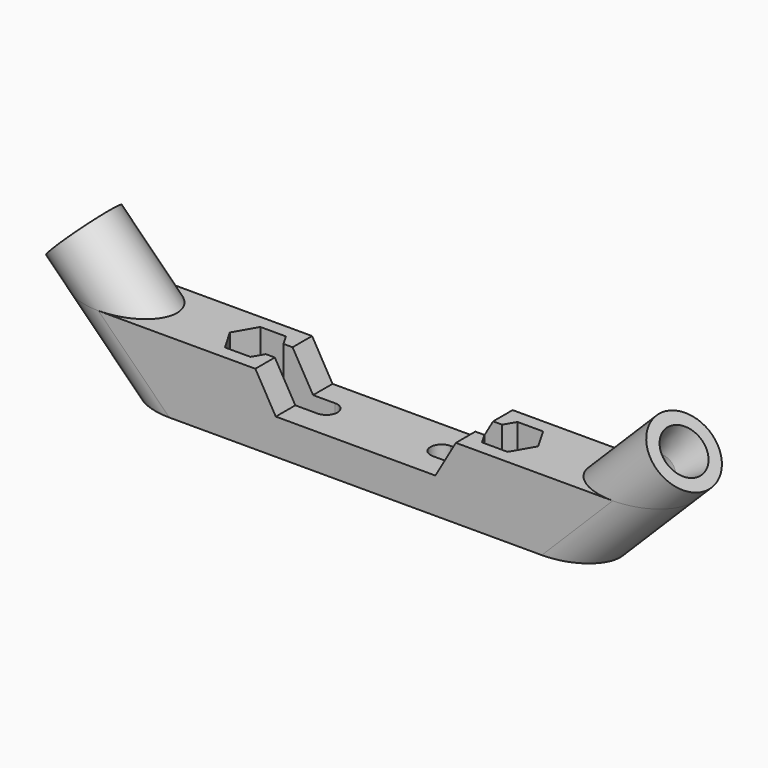
from build123d import *

# Parameters (mm, degrees)
F1_DEPTH  = 4
F2_R      = 3.99999
F4_DEPTH  = 8
F6_DEPTH  = 12.5
F9_R      = 4
F10_DEPTH = 6.851053331
F12_SIZE2 = 1
F12_SIZE  = 3.7320508076
F14_DEPTH = 8.001


# Not quite as in the source:
# - a fillet or chamfer is up to 0.001 mm smaller than in the source, because OpenCascade refuses the exact size


with BuildPart() as f1:
    # F0 (on Front) → F1 (new body, symmetric)
    with BuildSketch(Plane.XZ):
        Polygon((-26.6568542495, 0), (0, 0), (0, 8), (-34.6568542495, 8), align=None)
    extrude(amount=F1_DEPTH, both=True)

    # F2 (radius 4 in the source; OpenCascade refuses exactly that, so slightly less here)
    f2_edges = [f1.edges().sort_by_distance(p)[0] for p in [
        (-30.656854, 4, 4),
        (-30.656854, -4, 4),
    ]]
    fillet(f2_edges, radius=F2_R)

    # F3 (on face) → F4 (cut, through all)
    with BuildSketch(Plane.XY.offset(8)):
        Polygon((-11.6132486541, 0), (-13.056624327, 2.5), (-15.943375673, 2.5), (-17.3867513459, 0), (-15.943375673, -2.5), (-13.056624327, -2.5), align=None)
    extrude(amount=-F4_DEPTH, mode=Mode.SUBTRACT)

    # F5 (on Front) → F6 (cut, symmetric)
    with BuildSketch(Plane.XZ):
        Polygon((0, 4), (0, 11.6737775235), (-13.4304575189, 11.6737775235), (-9, 4), align=None)
    extrude(amount=F6_DEPTH, both=True, mode=Mode.SUBTRACT)

    # F9 (on line) → F10 (join, symmetric)
    with BuildSketch(Plane(origin=(-18.5, 0, 18.5), x_dir=(0, 1, 0), z_dir=(0.7071067812, 0, -0.7071067812))):
        with Locations((0, -14.8492424049)):
            Circle(F9_R)
    extrude(amount=F10_DEPTH, both=True)

    # F7 (on Front) → F11 (revolve, cut)
    with BuildSketch(Plane.XZ):
        Polygon((-11.4302859145, -11.8147781158), (-10.3077538993, -10.6922461007), (-44.6173825807, 23.6173825807), (-45.7399145958, 22.4948505656), align=None)
    revolve(axis=Axis((-27.46256824, 0, 6.46256824), (-0.7071067812, 0, 0.7071067812)), mode=Mode.SUBTRACT)

    # F12
    f12_edges = [f1.edges().sort_by_distance(p)[0] for p in [
        (-32.721894, 0, 13.966958),
    ]]
    f12_side = f1.faces().sort_by_distance((-25.685621, 0, 6.930685))[0]
    chamfer(f12_edges, length=F12_SIZE, length2=F12_SIZE2, reference=f12_side)

    # F13 (on face) → F14 (cut, through all)
    with BuildSketch(Plane.XY.offset(8)):
        with BuildLine():
            ThreePointArc((-14.5, 1.25), (-15.75, 0), (-14.5, -1.25))
            Line((-14.5, -1.25), (-6.5, -1.25))
            ThreePointArc((-6.5, -1.25), (-5.25, 0), (-6.5, 1.25))
            Line((-6.5, 1.25), (-14.5, 1.25))
        make_face()
    extrude(amount=-F14_DEPTH, mode=Mode.SUBTRACT)

    # F15: F1 across face


with BuildPart() as f1_1:
    add(f1.part)
    add(f1.part.mirror(Plane(origin=(0, 0, 2), x_dir=(0, 1, 0), z_dir=(1, 0, 0))))


solid = f1_1.part
